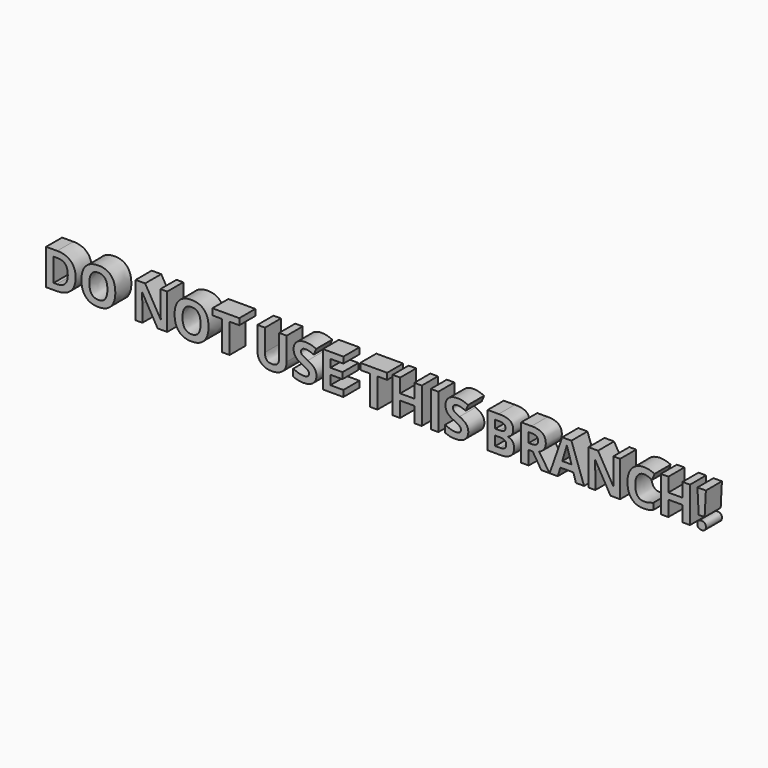
from build123d import *

# Parameters (mm, degrees)
F0_TEXT_SIZE = 24.8584430665
F1_DEPTH     = 10


# Not quite as in the source:
# - Text() gives the source's letters only with a copy of the font that has no kerning and outlines rounded to 1/6400 em; it was checked with that copy


with BuildPart() as f1:
    # F0 (on Front) → F1 (new body)
    with BuildSketch(Plane.XZ):
        with Locations((-145.3135460615, 35.0871197879)):
            Text('DO NOT USE THIS BRANCH!', F0_TEXT_SIZE, font='Open Sans', font_style=FontStyle.BOLD, text_align=(TextAlign.LEFT, TextAlign.BOTTOM))
    extrude(amount=F1_DEPTH)


solid = f1.part
